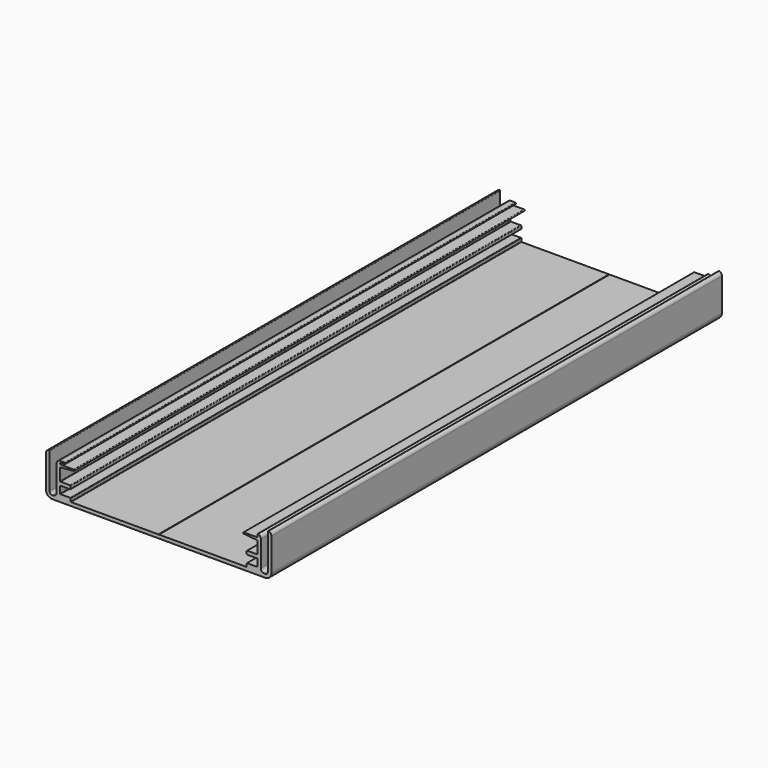
from build123d import *

# Parameters (mm, degrees)
F1_DEPTH = 508


# Not quite as in the source:
# - ends of sketch curves that miss each other by under 0.0002 mm in the source are joined


with BuildPart() as f1:
    # F0 (on Front) → F1 (new body)
    with BuildSketch(Plane.XZ):
        with BuildLine():
            Line((-125.4417608, 32.418528), (-110.7097608, 32.418528))
            Line((-110.7097608, 32.418528), (-110.3287608, 32.799528))
            Line((-110.3287608, 32.799528), (-109.9477608, 32.418528))
            Line((-109.9477608, 32.418528), (51.1898392, 32.418528))
            Line((51.1898392, 32.418528), (51.5708392, 32.799528))
            Line((51.5708392, 32.799528), (51.9518392, 32.418528))
            Line((51.9518392, 32.418528), (66.6838392, 32.418528))
            ThreePointArc((66.6838392, 32.418528), (70.5992308688, 34.0403363312), (72.2210392, 37.955728))
            Line((72.2210392, 37.955728), (72.2210392, 67.4102538))
            ThreePointArc((72.2210392, 67.4102538), (71.5313659528, 69.3860513433), (69.7619677468, 70.5034837164))
            ThreePointArc((69.7619677468, 70.5034837164), (69.2666914482, 70.3916273244), (69.0460392, 69.934328))
            Line((69.0460392, 69.934328), (69.0460392, 37.955728))
            ThreePointArc((69.0460392, 37.955728), (68.3541668385, 36.2854003615), (66.6838392, 35.593528))
            Line((66.6838392, 35.593528), (65.8710392, 35.593528))
            ThreePointArc((65.8710392, 35.593528), (63.6259751697, 36.5234639697), (62.6960392, 38.768528))
            Line((62.6960392, 38.768528), (62.6960392, 62.0254538))
            ThreePointArc((62.6960392, 62.0254538), (62.0063659528, 64.0012513433), (60.2369677468, 65.1186837164))
            ThreePointArc((60.2369677468, 65.1186837164), (59.7416914482, 65.0068273244), (59.5210392, 64.549528))
            Line((59.5210392, 64.549528), (59.5210392, 62.644528))
            ThreePointArc((59.5210392, 62.644528), (59.4094468836, 62.3751203164), (59.1400392, 62.263528))
            Line((59.1400392, 62.263528), (47.4052392, 62.263528))
            ThreePointArc((47.4052392, 62.263528), (46.8216542466, 61.706128041), (47.3516955482, 61.0975868915))
            Line((47.3516955482, 61.0975868915), (58.9903824, 60.0263722))
            ThreePointArc((58.9903824, 60.0263722), (59.3684465687, 59.8383423872), (59.5210392, 59.444636))
            Line((59.5210392, 59.444636), (59.5210392, 49.055528))
            ThreePointArc((59.5210392, 49.055528), (59.4094468836, 48.7861203164), (59.1400392, 48.674528))
            Line((59.1400392, 48.674528), (50.5802392, 48.674528))
            ThreePointArc((50.5802392, 48.674528), (50.1671474184, 48.5034197816), (49.9960392, 48.090328))
            Line((49.9960392, 48.090328), (49.9960392, 46.083728))
            ThreePointArc((49.9960392, 46.083728), (50.1671474184, 45.6706362184), (50.5802392, 45.499528))
            Line((50.5802392, 45.499528), (59.1400392, 45.499528))
            ThreePointArc((59.1400392, 45.499528), (59.4094468836, 45.3879356836), (59.5210392, 45.118528))
            Line((59.5210392, 45.118528), (59.5210392, 39.149528))
            ThreePointArc((59.5210392, 39.149528), (59.4094468836, 38.8801203164), (59.1400392, 38.768528))
            Line((59.1400392, 38.768528), (50.3770392, 38.768528))
            ThreePointArc((50.3770392, 38.768528), (50.1076315164, 38.6569356836), (49.9960392, 38.387528))
            Line((49.9960392, 38.387528), (49.9960392, 35.974528))
            ThreePointArc((49.9960392, 35.974528), (49.8844468836, 35.7051203164), (49.6150392, 35.593528))
            Line((49.6150392, 35.593528), (-29.1249608, 35.593528))
            Line((-29.1249608, 35.593528), (-29.3789608, 35.339528))
            Line((-29.3789608, 35.339528), (-29.6329608, 35.593528))
            Line((-29.6329608, 35.593528), (-108.3729608, 35.593528))
            ThreePointArc((-108.3729608, 35.593528), (-108.6423684836, 35.7051203164), (-108.7539608, 35.974528))
            Line((-108.7539608, 35.974528), (-108.7539608, 38.387528))
            ThreePointArc((-108.7539608, 38.387528), (-108.8655531164, 38.6569356836), (-109.1349608, 38.768528))
            Line((-109.1349608, 38.768528), (-117.8979608, 38.768528))
            ThreePointArc((-117.8979608, 38.768528), (-118.1673684836, 38.8801203164), (-118.2789608, 39.149528))
            Line((-118.2789608, 39.149528), (-118.2789608, 45.118528))
            ThreePointArc((-118.2789608, 45.118528), (-118.1673684836, 45.3879356836), (-117.8979608, 45.499528))
            Line((-117.8979608, 45.499528), (-109.3381608, 45.499528))
            ThreePointArc((-109.3381608, 45.499528), (-108.9250690184, 45.6706362184), (-108.7539608, 46.083728))
            Line((-108.7539608, 46.083728), (-108.7539608, 48.090328))
            ThreePointArc((-108.7539608, 48.090328), (-108.9250690184, 48.5034197816), (-109.3381608, 48.674528))
            Line((-109.3381608, 48.674528), (-117.8979608, 48.674528))
            ThreePointArc((-117.8979608, 48.674528), (-118.1673684836, 48.7861203164), (-118.2789608, 49.055528))
            Line((-118.2789608, 49.055528), (-118.2789608, 59.444636))
            ThreePointArc((-118.2789608, 59.444636), (-118.1263681687, 59.8383423872), (-117.7483044518, 60.0263771085))
            Line((-117.7483044518, 60.0263771085), (-106.1096176, 61.0975918))
            ThreePointArc((-106.1096176, 61.0975918), (-105.5795758466, 61.706128041), (-106.1631608, 62.263528))
            Line((-106.1631608, 62.263528), (-117.4788608, 62.263528))
            ThreePointArc((-117.4788608, 62.263528), (-118.0446169356, 62.4978718644), (-118.2789608, 63.063628))
            ThreePointArc((-118.2789608, 63.063628), (-118.0446169356, 63.6293841356), (-117.4788608, 63.863728))
            Line((-117.4788608, 63.863728), (-114.1387608, 63.863728))
            ThreePointArc((-114.1387608, 63.863728), (-113.6897479939, 64.0497151939), (-113.5037608, 64.498728))
            ThreePointArc((-113.5037608, 64.498728), (-113.6897479939, 64.9477408061), (-114.1387608, 65.133728))
            Line((-114.1387608, 65.133728), (-118.2789608, 65.133728))
            ThreePointArc((-118.2789608, 65.133728), (-120.5240248303, 64.2037920303), (-121.4539608, 61.958728))
            Line((-121.4539608, 61.958728), (-121.4539608, 38.768528))
            ThreePointArc((-121.4539608, 38.768528), (-122.3838967697, 36.5234639697), (-124.6289608, 35.593528))
            Line((-124.6289608, 35.593528), (-125.4417608, 35.593528))
            ThreePointArc((-125.4417608, 35.593528), (-127.1120884385, 36.2854003615), (-127.8039608, 37.955728))
            Line((-127.8039608, 37.955728), (-127.8039608, 69.934328))
            ThreePointArc((-127.8039608, 69.934328), (-128.0246130482, 70.3916273244), (-128.5198891538, 70.503482883))
            ThreePointArc((-128.5198891538, 70.503482883), (-130.2892875528, 69.3860513433), (-130.9789608, 67.4102538))
            Line((-130.9789608, 67.4102538), (-130.9789608, 37.955728))
            ThreePointArc((-130.9789608, 37.955728), (-129.3571524688, 34.0403363312), (-125.4417608, 32.418528))
        make_face()
    extrude(amount=F1_DEPTH)


solid = f1.part
